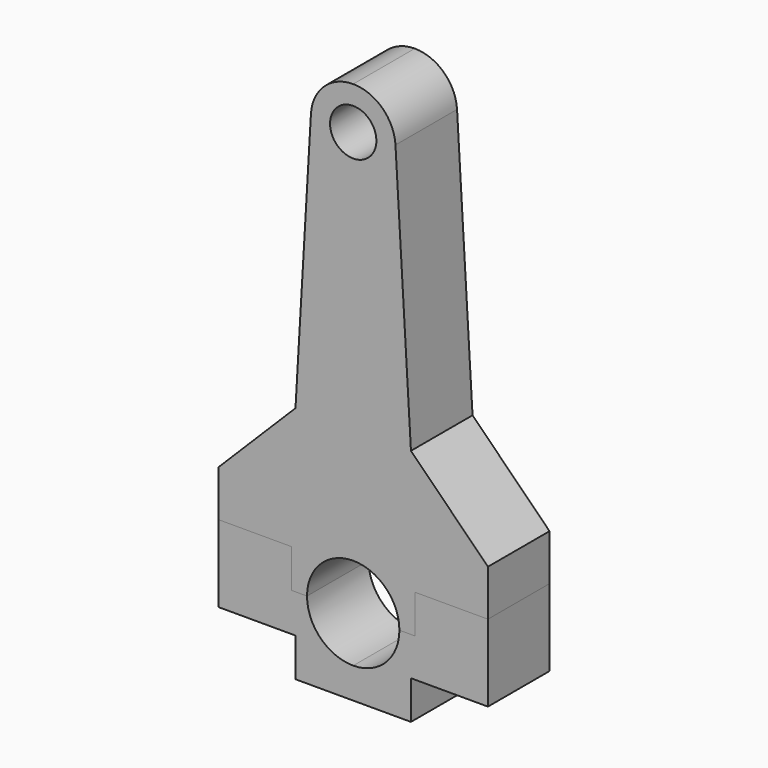
from build123d import *

# Parameters (mm, degrees)
F1_DEPTH      = 5
F2_R          = 2.1
F3_DEPTH      = 12.5
F6_DEPTH      = 5
F6_DEPTH_BACK = 5
F8_D          = 3.3
F8_DEPTH      = 9
F8_TIP        = 0.9914200214


with BuildPart() as f1:
    # F0 (on Front) → F1 (new body, symmetric)
    with BuildSketch(Plane.XZ):
        with BuildLine():
            ThreePointArc((0, -6), (-4.2426406871, -4.2426406871), (-6, 0))
            Line((-6, 0), (-8, 0))
            Line((-8, 0), (-8, 5))
            Line((-8, 5), (-17.5, 5))
            Line((-17.5, 5), (-17.5, -5))
            Line((-17.5, -5), (-7.5, -5))
            Line((-7.5, -5), (-7.5, -10))
            Line((-7.5, -10), (0, -10))
            Line((0, -10), (0, -6))
        make_face()
    extrude(amount=F1_DEPTH, both=True)

    # F2 (on Top) → F3 (cut, symmetric)
    with BuildSketch(Plane.XY):
        with Locations((-12.75, 0)):
            Circle(F2_R)
    extrude(amount=F3_DEPTH, both=True, mode=Mode.SUBTRACT)

    # F4: F1 across plane


with BuildPart() as f1_1:
    add(f1.part)
    add(f1.part.mirror(Plane.YZ))


with BuildPart() as f6:
    # F5 (on Front) → F6 (new body, two sides)
    with BuildSketch(Plane.XZ) as f6_sk:
        with BuildLine():
            Line((-8, 0), (-6, 0))
            ThreePointArc((-6, 0), (-4.2426406871, 4.2426406871), (0, 6))
            Line((0, 6), (0, 51.99))
            ThreePointArc((0, 51.99), (-3.01, 55), (0, 58.01))
            Line((0, 58.01), (0, 60.5))
            ThreePointArc((0, 60.5), (-3.7737246239, 59.0011251497), (-5.4905980002, 55.3214554412))
            Line((-5.4905980002, 55.3214554412), (-7.5, 21))
            Line((-7.5, 21), (-17.5, 11))
            Line((-17.5, 11), (-17.5, 5))
            Line((-17.5, 5), (-8, 5))
            Line((-8, 5), (-8, 0))
        make_face()
    extrude(amount=F6_DEPTH)
    extrude(f6_sk.sketch, amount=-F6_DEPTH_BACK)

    # F8
    with Locations(Plane(origin=(0, 0, 5), x_dir=(1, 0, 0), z_dir=(0, 0, -1))):
        with Locations((-12.75, 0)):
            Hole(F8_D / 2, depth=F8_DEPTH)
            with Locations((0, 0, -(F8_DEPTH + F8_TIP / 2))):  # 118° drill point
                Cone(0, F8_D / 2, F8_TIP, mode=Mode.SUBTRACT)

    # F9: F6 across plane


with BuildPart() as f6_1:
    add(f6.part)
    add(f6.part.mirror(Plane.YZ))


solid = Compound([f1_1.part, f6_1.part])
